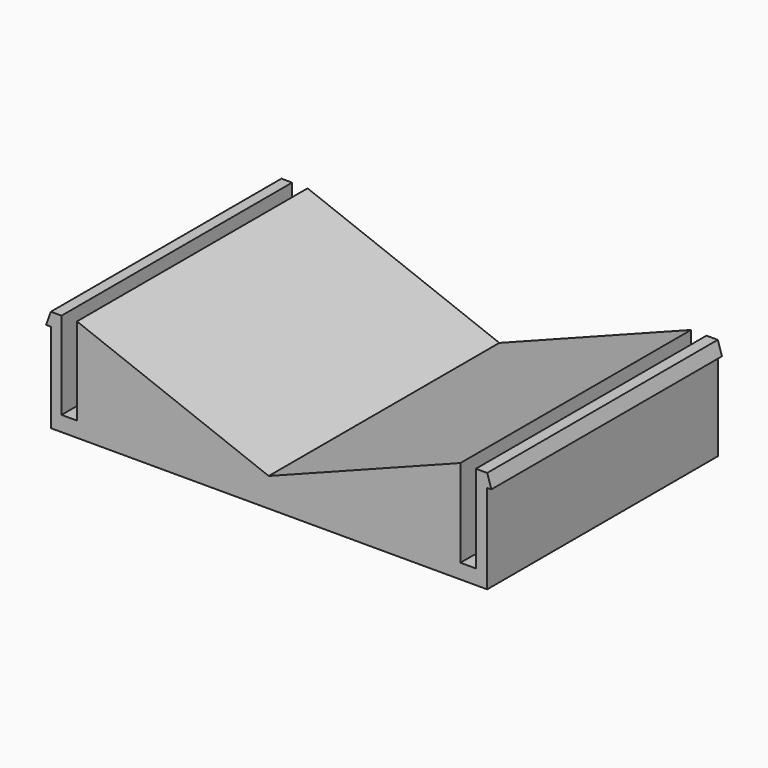
from build123d import *

# Parameters (mm, degrees)
F0_W     = 6.64972
F0_H     = 4.99872
F1_DEPTH = 1.778
F3_DEPTH = 25.4
F4_W     = 0.26797
F4_H     = 1.5150946512
F4_H_2   = 0.2629053488
F4_H_3   = 0.255633
F4_H_4   = 1.522367
F5_DEPTH = 4.99872
F6_W     = 0.0717422777
F6_H     = 1.5494
F6_W_2   = 0.0822888074
F7_DEPTH = 25.4


with BuildPart() as f1:
    # F0 (on Top) → F1 (new body)
    with BuildSketch(Plane.XY):
        with Locations((0, 0.1761515194)):
            Rectangle(F0_W, F0_H)
    extrude(amount=F1_DEPTH)

    # F2 (on face) → F3 (cut)
    with BuildSketch(Plane.XZ.offset(2.3232084806)):
        Polygon((-3.32486, 1.778), (0, 0.4989000154), (3.32486, 1.778), align=None)
    extrude(amount=-F3_DEPTH, mode=Mode.SUBTRACT)

    # F4 (on face) → F5 (join, through all)
    with BuildSketch(Plane.XZ.offset(2.3232084806)):
        with Locations((-3.726815, 1.0204526744)):
            Rectangle(F4_W, F4_H)
        with Locations((-3.726815, 0.1314526744)):
            Rectangle(F4_W, F4_H_2)
        with Locations((-3.458845, 0.1314526744)):
            Rectangle(F4_W, F4_H_2)
        with Locations((3.458845, 0.1278165)):
            Rectangle(F4_W, F4_H_3)
        with Locations((3.726815, 0.1278165)):
            Rectangle(F4_W, F4_H_3)
        with Locations((3.726815, 1.0168165)):
            Rectangle(F4_W, F4_H_4)
    extrude(amount=-F5_DEPTH)

    # F6 (on face) → F7 (cut)
    with BuildSketch(Plane(origin=(0, 2.6755115194, 0), x_dir=(-1, 0, 0), z_dir=(0, 1, 0))):
        with Locations((-3.8249288612, 0.7747)):
            Rectangle(F6_W, F6_H)
        Polygon((-3.8608, 1.778), (-3.8608, 1.5494), (-3.7890577223, 1.778), align=None)
        Polygon((3.7785111926, 1.778), (3.8608, 1.5494), (3.8608, 1.778), align=None)
        with Locations((3.8196555963, 0.7747)):
            Rectangle(F6_W_2, F6_H)
    extrude(amount=-F7_DEPTH, mode=Mode.SUBTRACT)


solid = f1.part
